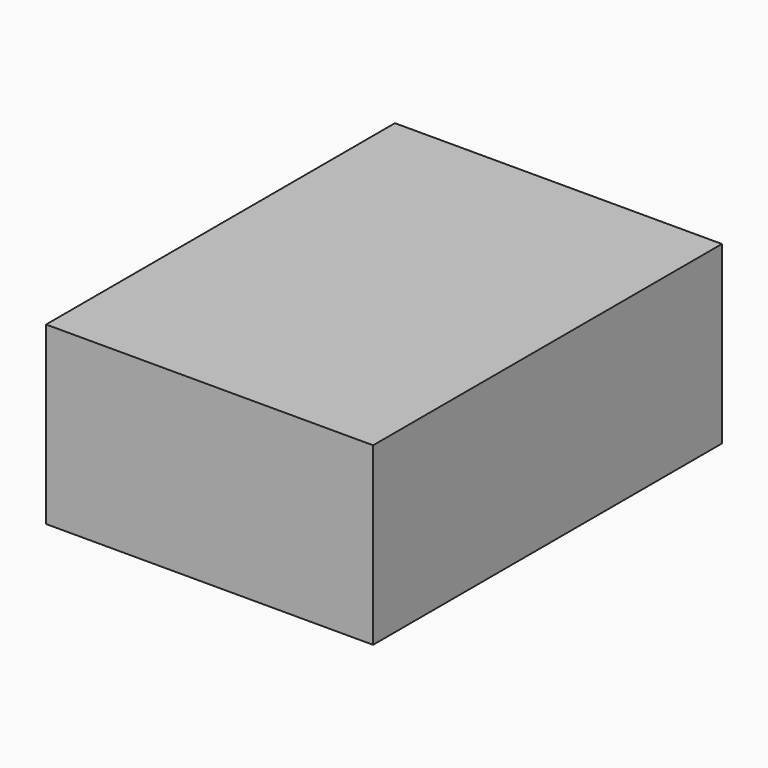
from build123d import *

# Parameters (mm, degrees)
F0_W         = 76.2
F0_H         = 101.6
F1_DEPTH     = 38.1
F3_W         = 76.2
F3_H         = 101.6
F3_W_2       = 73.66
F3_H_2       = 99.06
F4_DEPTH     = 3.175
F5_T1_DEPTH  = 99.06
F5_T3_DEPTH  = 73.66
F5_T9_DEPTH  = 105.41
F5_T15_DEPTH = 80.01
F5_T24_DEPTH = 105.41
F5_T30_DEPTH = 80.01
F5_T39_DEPTH = 80.01
F5_T45_DEPTH = 105.41
F5_T54_DEPTH = 105.41
F5_T60_DEPTH = 80.01


# Not quite as in the source:
# - a fillet or chamfer that OpenCascade refuses, or shapes differently, is made with other operations: its cross-section is extruded or revolved along the edge and cut away or added


with BuildPart() as f1:
    # F0 (on Top) → F1 (new body)
    with BuildSketch(Plane.XY):
        Rectangle(F0_W, F0_H)
    extrude(amount=F1_DEPTH)

    # F3 (on face) → F4 (join)
    with BuildSketch(Plane(origin=(0, 0, 0), x_dir=(1, 0, 0), z_dir=(0, 0, -1))):
        Rectangle(F3_W, F3_H)
        Rectangle(F3_W_2, F3_H_2, mode=Mode.SUBTRACT)
    extrude(amount=F4_DEPTH)

    # F5: fillet of radius 2.54 on 4 edges, made by hand

    # F5_s2 → F5_t1 (cut)
    with BuildSketch(Plane.XZ.offset(-49.53)):
        with BuildLine():
            ThreePointArc((-39.37, -3.175), (-37.5739487758, -2.4310512242), (-36.83, -0.635))
            Line((-36.83, -0.635), (-36.83, -3.175))
            Line((-36.83, -3.175), (-39.37, -3.175))
        make_face()
        with BuildLine():
            ThreePointArc((39.37, -3.175), (37.5739487758, -2.4310512242), (36.83, -0.635))
            Line((36.83, -0.635), (36.83, -3.175))
            Line((36.83, -3.175), (39.37, -3.175))
        make_face()
    extrude(amount=F5_T1_DEPTH, mode=Mode.SUBTRACT)

    # F5_s4 → F5_t3 (cut)
    with BuildSketch(Plane.YZ.offset(-36.83)):
        with BuildLine():
            ThreePointArc((-52.07, -3.175), (-50.2739487758, -2.4310512242), (-49.53, -0.635))
            Line((-49.53, -0.635), (-49.53, -3.175))
            Line((-49.53, -3.175), (-52.07, -3.175))
        make_face()
        with BuildLine():
            ThreePointArc((52.07, -3.175), (50.2739487758, -2.4310512242), (49.53, -0.635))
            Line((49.53, -0.635), (49.53, -3.175))
            Line((49.53, -3.175), (52.07, -3.175))
        make_face()
    extrude(amount=F5_T3_DEPTH, mode=Mode.SUBTRACT)


with BuildPart() as f5_tool7:
    # F5_s8 → F5_t9 (new body)
    with BuildSketch(Plane.XZ.offset(-55.88)):
        with BuildLine():
            ThreePointArc((-39.37, -3.175), (-37.5739487758, -2.4310512242), (-36.83, -0.635))
            Line((-36.83, -0.635), (-36.83, -3.175))
            Line((-36.83, -3.175), (-39.37, -3.175))
        make_face()
    extrude(amount=F5_T9_DEPTH)

    split(bisect_by=Plane.XZ.offset(-49.53), keep=Keep.BOTTOM)

    split(bisect_by=Plane.YZ.offset(-38.1), keep=Keep.TOP)

    split(bisect_by=Plane.XZ.offset(-50.8), keep=Keep.TOP)


with BuildPart() as f5_tool13:
    # F5_s14 → F5_t15 (new body)
    with BuildSketch(Plane.YZ.offset(36.83)):
        with BuildLine():
            ThreePointArc((52.07, -3.175), (50.2739487758, -2.4310512242), (49.53, -0.635))
            Line((49.53, -0.635), (49.53, -3.175))
            Line((49.53, -3.175), (52.07, -3.175))
        make_face()
    extrude(amount=-F5_T15_DEPTH)

    split(bisect_by=Plane.YZ.offset(-36.83), keep=Keep.BOTTOM)

    split(bisect_by=Plane.YZ.offset(-38.1), keep=Keep.TOP)

    split(bisect_by=Plane.XZ.offset(-50.8), keep=Keep.TOP)


with BuildPart() as f5_tool7_1:
    add(f5_tool7.part)

    # F5_t19: intersect F5_tool13
    add(f5_tool13.part, mode=Mode.INTERSECT)


with BuildPart() as f1_1:
    add(f1.part)

    # F5_t5: cut F5_tool7
    add(f5_tool7_1.part, mode=Mode.SUBTRACT)


with BuildPart() as f5_tool22:
    # F5_s23 → F5_t24 (new body)
    with BuildSketch(Plane.XZ.offset(-49.53)):
        with BuildLine():
            ThreePointArc((-39.37, -3.175), (-37.5739487758, -2.4310512242), (-36.83, -0.635))
            Line((-36.83, -0.635), (-36.83, -3.175))
            Line((-36.83, -3.175), (-39.37, -3.175))
        make_face()
    extrude(amount=F5_T24_DEPTH)

    split(bisect_by=Plane.XZ.offset(49.53), keep=Keep.TOP)

    split(bisect_by=Plane.YZ.offset(-38.1), keep=Keep.TOP)

    split(bisect_by=Plane.XZ.offset(50.8), keep=Keep.BOTTOM)


with BuildPart() as f5_tool28:
    # F5_s29 → F5_t30 (new body)
    with BuildSketch(Plane.YZ.offset(-43.18)):
        with BuildLine():
            ThreePointArc((-52.07, -3.175), (-50.2739487758, -2.4310512242), (-49.53, -0.635))
            Line((-49.53, -0.635), (-49.53, -3.175))
            Line((-49.53, -3.175), (-52.07, -3.175))
        make_face()
    extrude(amount=F5_T30_DEPTH)

    split(bisect_by=Plane.YZ.offset(-36.83), keep=Keep.BOTTOM)

    split(bisect_by=Plane.YZ.offset(-38.1), keep=Keep.TOP)

    split(bisect_by=Plane.XZ.offset(50.8), keep=Keep.BOTTOM)


with BuildPart() as f5_tool22_1:
    add(f5_tool22.part)

    # F5_t34: intersect F5_tool28
    add(f5_tool28.part, mode=Mode.INTERSECT)


with BuildPart() as f1_2:
    add(f1_1.part)

    # F5_t20: cut F5_tool22
    add(f5_tool22_1.part, mode=Mode.SUBTRACT)


with BuildPart() as f5_tool37:
    # F5_s38 → F5_t39 (new body)
    with BuildSketch(Plane.YZ.offset(-36.83)):
        with BuildLine():
            ThreePointArc((-52.07, -3.175), (-50.2739487758, -2.4310512242), (-49.53, -0.635))
            Line((-49.53, -0.635), (-49.53, -3.175))
            Line((-49.53, -3.175), (-52.07, -3.175))
        make_face()
    extrude(amount=F5_T39_DEPTH)

    split(bisect_by=Plane.YZ.offset(38.1), keep=Keep.BOTTOM)

    split(bisect_by=Plane.YZ.offset(36.83), keep=Keep.TOP)

    split(bisect_by=Plane.XZ.offset(50.8), keep=Keep.BOTTOM)


with BuildPart() as f5_tool43:
    # F5_s44 → F5_t45 (new body)
    with BuildSketch(Plane.XZ.offset(55.88)):
        with BuildLine():
            ThreePointArc((39.37, -3.175), (37.5739487758, -2.4310512242), (36.83, -0.635))
            Line((36.83, -0.635), (36.83, -3.175))
            Line((36.83, -3.175), (39.37, -3.175))
        make_face()
    extrude(amount=-F5_T45_DEPTH)

    split(bisect_by=Plane.YZ.offset(38.1), keep=Keep.BOTTOM)

    split(bisect_by=Plane.XZ.offset(49.53), keep=Keep.TOP)

    split(bisect_by=Plane.XZ.offset(50.8), keep=Keep.BOTTOM)


with BuildPart() as f5_tool37_1:
    add(f5_tool37.part)

    # F5_t49: intersect F5_tool43
    add(f5_tool43.part, mode=Mode.INTERSECT)


with BuildPart() as f1_3:
    add(f1_2.part)

    # F5_t35: cut F5_tool37
    add(f5_tool37_1.part, mode=Mode.SUBTRACT)


with BuildPart() as f5_tool52:
    # F5_s53 → F5_t54 (new body)
    with BuildSketch(Plane.XZ.offset(49.53)):
        with BuildLine():
            ThreePointArc((39.37, -3.175), (37.5739487758, -2.4310512242), (36.83, -0.635))
            Line((36.83, -0.635), (36.83, -3.175))
            Line((36.83, -3.175), (39.37, -3.175))
        make_face()
    extrude(amount=-F5_T54_DEPTH)

    split(bisect_by=Plane.YZ.offset(38.1), keep=Keep.BOTTOM)

    split(bisect_by=Plane.XZ.offset(-49.53), keep=Keep.BOTTOM)

    split(bisect_by=Plane.XZ.offset(-50.8), keep=Keep.TOP)


with BuildPart() as f5_tool58:
    # F5_s59 → F5_t60 (new body)
    with BuildSketch(Plane.YZ.offset(43.18)):
        with BuildLine():
            ThreePointArc((52.07, -3.175), (50.2739487758, -2.4310512242), (49.53, -0.635))
            Line((49.53, -0.635), (49.53, -3.175))
            Line((49.53, -3.175), (52.07, -3.175))
        make_face()
    extrude(amount=-F5_T60_DEPTH)

    split(bisect_by=Plane.YZ.offset(38.1), keep=Keep.BOTTOM)

    split(bisect_by=Plane.YZ.offset(36.83), keep=Keep.TOP)

    split(bisect_by=Plane.XZ.offset(-50.8), keep=Keep.TOP)


with BuildPart() as f5_tool52_1:
    add(f5_tool52.part)

    # F5_t64: intersect F5_tool58
    add(f5_tool58.part, mode=Mode.INTERSECT)


with BuildPart() as f1_4:
    add(f1_3.part)

    # F5_t50: cut F5_tool52
    add(f5_tool52_1.part, mode=Mode.SUBTRACT)


solid = f1_4.part
